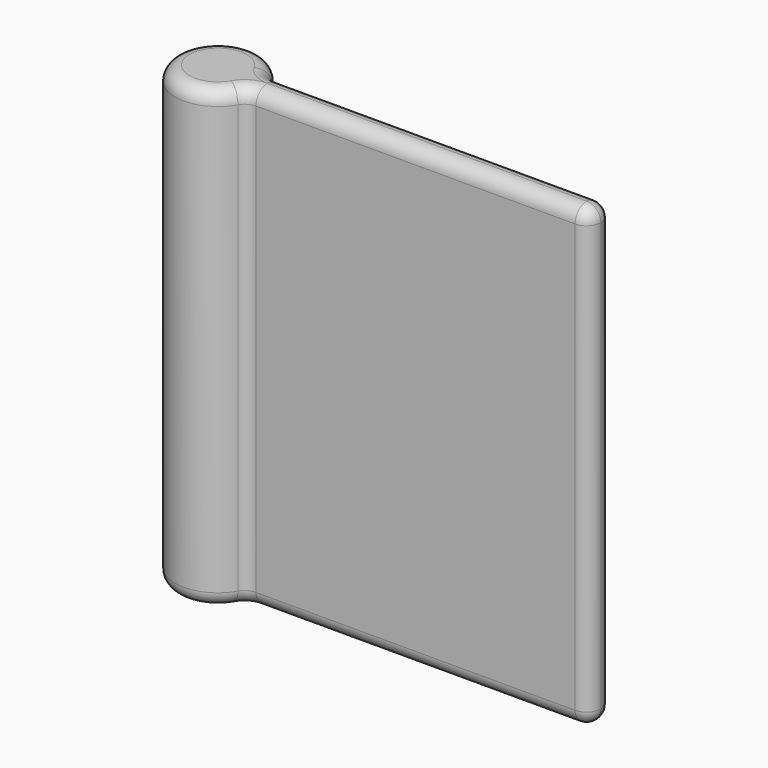
from build123d import *

# Parameters (mm, degrees)
F1_DEPTH = 25.4
F2_R     = 0.79374


# Not quite as in the source:
# - a fillet or chamfer is up to 0.001 mm smaller than in the source, because OpenCascade refuses the exact size
# - a feature names something its author has since deleted; it is built from what else it names


with BuildPart() as f1:
    # F0 (on Top) → F1 (new body)
    with BuildSketch(Plane.XY):
        with BuildLine():
            ThreePointArc((2.2450640303, -0.79375), (2.3469565702, -0.4026740868), (2.38125, 0))
            ThreePointArc((2.38125, 0), (2.3469565702, 0.4026740868), (2.2450640303, 0.79375))
            ThreePointArc((2.2450640303, 0.79375), (-2.38125, 0), (2.2450640303, -0.79375))
        make_face()
        with BuildLine():
            ThreePointArc((2.2450640303, 0.79375), (2.3469565702, 0.4026740868), (2.38125, 0))
            ThreePointArc((2.38125, 0), (2.3469565702, -0.4026740868), (2.2450640303, -0.79375))
            Line((2.2450640303, -0.79375), (21.2950640303, -0.79375))
            Line((21.2950640303, -0.79375), (21.2950640303, 0))
            Line((21.2950640303, 0), (21.2950640303, 0.79375))
            Line((21.2950640303, 0.79375), (2.2450640303, 0.79375))
        make_face()
    extrude(amount=F1_DEPTH)

    # F2 (radius 0.79375 in the source; OpenCascade refuses exactly that, so slightly less here)
    f2_edges = [f1.edges().sort_by_distance(p)[0] for p in [
        (-2.38125, 0, 25.4),
        (11.770064, -0.79375, 25.4),
        (21.295064, 0, 25.4),
        (11.770064, 0.79375, 25.4),
        (-2.38125, 0, 0),
        (11.770064, -0.79375, 0),
        (21.295064, 0, 0),
        (11.770064, 0.79375, 0),
        (21.295064, 0.79375, 12.7),
        (2.245064, 0.79375, 12.7),
        (2.245064, -0.79375, 12.7),
        (21.295064, -0.79375, 12.7),
    ]]
    fillet(f2_edges, radius=F2_R)


solid = f1.part
